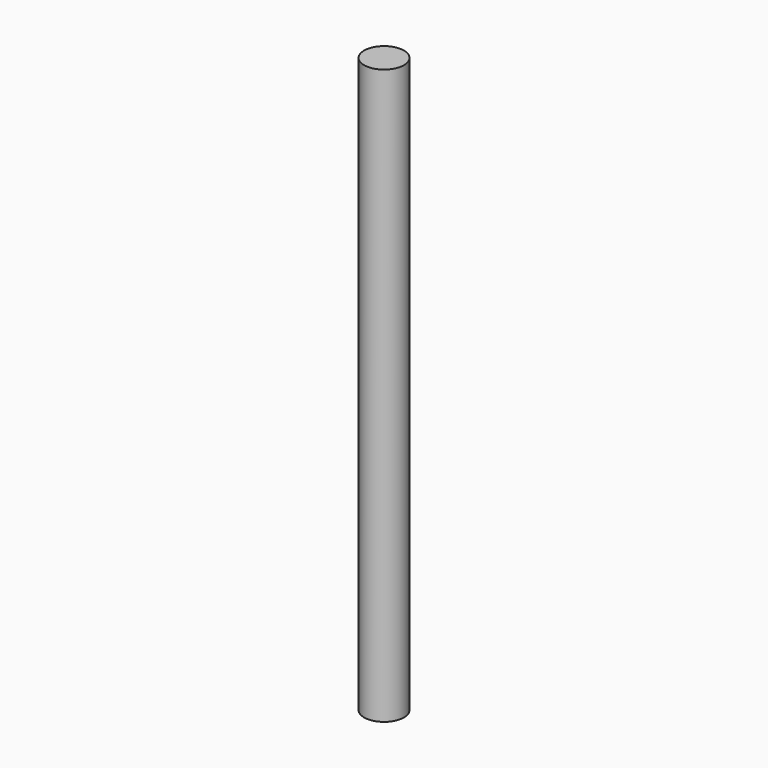
from build123d import *

# Parameters (mm, degrees)
F4_R     = 0.4406519
F5_DEPTH = 12.7204982564


# Not quite as in the source:
# - the program builds the solid bodies; features that only make, move or delete a surface that nothing else refers to are left out


with BuildPart() as f5:
    # F4 (on Top) → F5 (new body, through all)
    with BuildSketch(Plane.XY):
        Circle(F4_R)
    extrude(amount=-F5_DEPTH)


solid = f5.part
